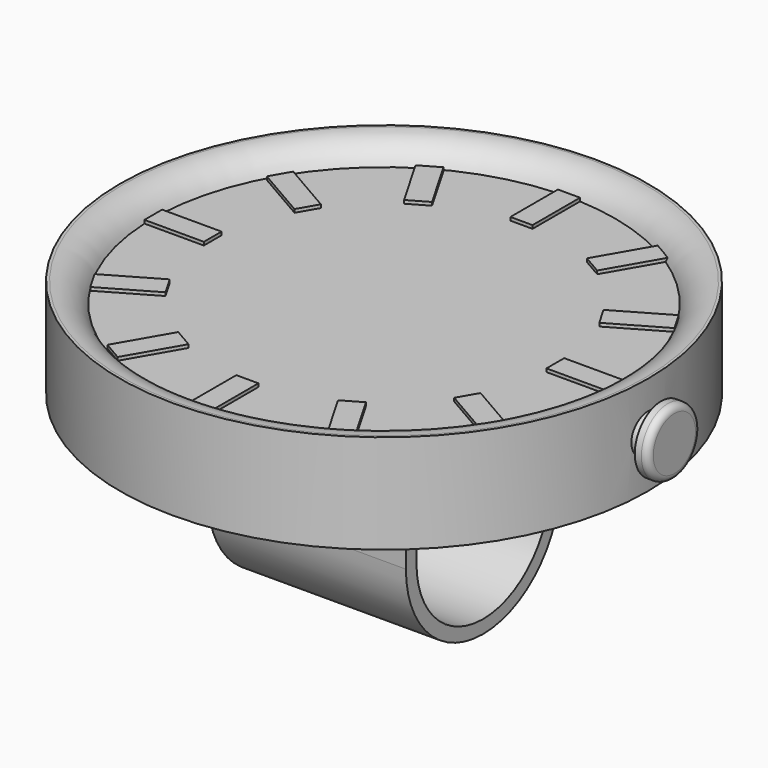
from build123d import *

# Parameters (mm, degrees)
F0_R      = 40
F0_R_2    = 35
F1_DEPTH  = 15
F2_R      = 35
F3_DEPTH  = 12
F5_R      = 3
F6_DEPTH  = 42
F7_R      = 5
F8_DEPTH  = 2
F9_R      = 1
F11_W     = 9
F11_H     = 3.350003619
F11_W_2   = 3.350003619
F11_H_2   = 9
F12_DEPTH = 0.5
F13_W     = 30
F13_H     = 2
F14_DEPTH = 12.6
F15_W     = 30
F15_H     = 2
F16_ANGLE = 180


# Not quite as in the source:
# - a fillet or chamfer that OpenCascade refuses, or shapes differently, is made with other operations: its cross-section is extruded or revolved along the edge and cut away or added


with BuildPart() as f1:
    # F0 (on Top) → F1 (new body)
    with BuildSketch(Plane.XY):
        Circle(F0_R)
        Circle(F0_R_2, mode=Mode.SUBTRACT)
    extrude(amount=F1_DEPTH)

    # F2 (on Top) → F3 (join)
    with BuildSketch(Plane.XY):
        Circle(F2_R)
    extrude(amount=F3_DEPTH)

    # F4: fillet of radius 5 on 1 edges, made by hand

    # F4_s1 → F4_t2 (revolve, cut)
    with BuildSketch(Plane.XZ):
        with BuildLine():
            ThreePointArc((39.582575695, 15), (36.8439629074, 14.1833001327), (35, 12))
            Line((35, 12), (35, 15))
            Line((35, 15), (39.582575695, 15))
        make_face()
    revolve(axis=Axis((0, 0, 15), (0, 0, 1)), mode=Mode.SUBTRACT)

    # F5 (on Right) → F6 (join)
    with BuildSketch(Plane.YZ):
        with Locations((0, 7.6651219279)):
            Circle(F5_R)
    extrude(amount=F6_DEPTH)

    # F7 (on face) → F8 (join)
    with BuildSketch(Plane.YZ.offset(42)):
        with Locations((0, 7.6651219279)):
            Circle(F7_R)
    extrude(amount=F8_DEPTH)

    # F9
    f9_edges = [f1.edges().sort_by_distance(p)[0] for p in [
        (44, -5, 7.665122),
    ]]
    fillet(f9_edges, radius=F9_R)

    # F11 (on face) → F12 (join)
    with BuildSketch(Plane.XY.offset(12)):
        with Locations((30.4598965808, 0)):
            Rectangle(F11_W, F11_H)
        with Locations((-30.4598965808, 0)):
            Rectangle(F11_W, F11_H)
        with Locations((0.064526599, 30.4573161602)):
            Rectangle(F11_W_2, F11_H_2)
        with Locations((0.064526599, -30.4573161602)):
            Rectangle(F11_W_2, F11_H_2)
        Polygon((29.9355077939, -18.884427597), (31.6105096033, -15.9832393602), (23.8162809693, -11.4832393602), (22.1412791598, -14.384427597), align=None)
        Polygon((-21.1475788678, 14.4766572205), (-28.9418075019, 18.9766572205), (-30.6168093114, 16.0754689837), (-22.8225806773, 11.5754689837), align=None)
        Polygon((19.4819840184, 29.4502744503), (16.5807957816, 31.1252762598), (12.0807957816, 23.3310476258), (14.9819840184, 21.6560458163), align=None)
        Polygon((-10.9753321418, -23.3033446013), (-13.8765203786, -21.6283427918), (-18.3765203786, -29.4225714259), (-15.4753321418, -31.0975732354), align=None)
        Polygon((31.3365066639, 15.8443492635), (29.6615048544, 18.7455375003), (21.8672762203, 14.2455375003), (23.5422780298, 11.3443492635), align=None)
        Polygon((-23.0965836168, -11.7143590805), (-30.8908122509, -16.2143590805), (-29.2158104414, -19.1155473173), (-21.4215818073, -14.6155473173), align=None)
        Polygon((-15.7493350812, 30.9586831386), (-18.650523318, 29.2836813291), (-14.150523318, 21.489452695), (-11.2493350812, 23.1644545045), align=None)
        Polygon((14.707981079, -21.7949359131), (11.8067928422, -23.4699377226), (16.3067928422, -31.2641663566), (19.207981079, -29.5891645471), align=None)
    extrude(amount=F12_DEPTH)

    # F13 (on face) → F14 (join)
    with BuildSketch(Plane(origin=(0, 0, 0), x_dir=(1, 0, 0), z_dir=(0, 0, -1))):
        with Locations((0, -13.6)):
            Rectangle(F13_W, F13_H)
        with Locations((0, 13.6)):
            Rectangle(F13_W, F13_H)
    extrude(amount=F14_DEPTH)

    # F15 (on face) → F16 (revolve)
    with BuildSketch(Plane(origin=(0, 0, -12.6), x_dir=(1, 0, 0), z_dir=(0, 0, -1))):
        with Locations((0, 13.6)):
            Rectangle(F15_W, F15_H)
    revolve(axis=Axis((9.313e-07, 0, -12.6), (1, 0, 0)), revolution_arc=F16_ANGLE)


solid = f1.part
